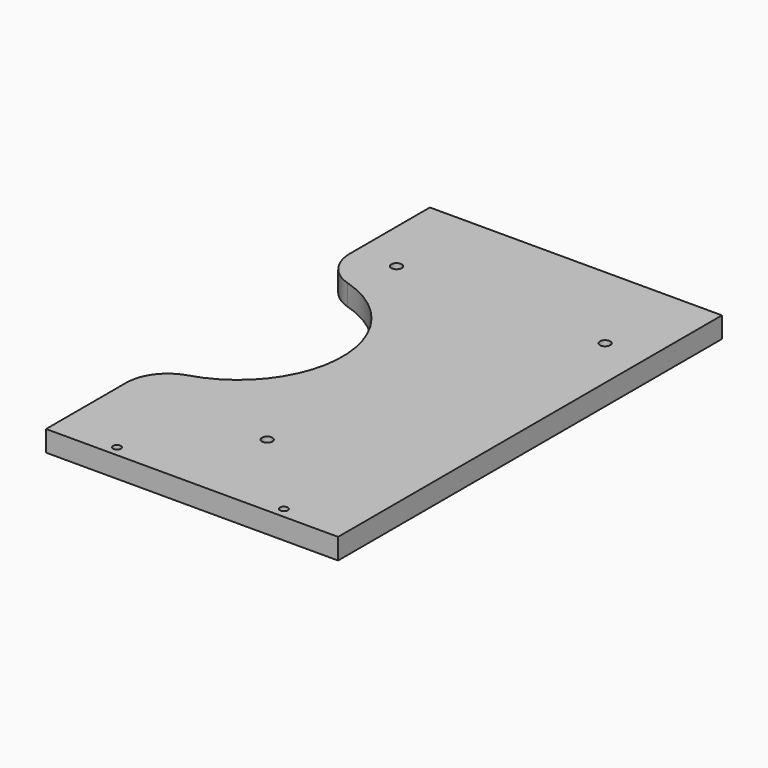
from build123d import *

# Parameters (mm, degrees)
F0_R     = 3.175
F1_DEPTH = 12.7
F2_R     = 25.4
F3_R     = 2.38125
F4_DEPTH = 12.701


with BuildPart() as f1:
    # F0 (on Top) → F1 (new body)
    with BuildSketch(Plane.XY):
        with BuildLine():
            Line((88.9, -146.05), (88.9, 146.05))
            Line((88.9, 146.05), (-88.9, 146.05))
            Line((-88.9, 146.05), (-88.9, 63.5))
            ThreePointArc((-88.9, 63.5), (-25.4, 0), (-88.9, -63.5))
            Line((-88.9, -63.5), (-88.9, -146.05))
            Line((-88.9, -146.05), (88.9, -146.05))
        make_face()
        with Locations((0, -88.9)):
            Circle(F0_R, mode=Mode.SUBTRACT)
        with Locations((-63.5, 88.9)):
            Circle(F0_R, mode=Mode.SUBTRACT)
        with Locations((63.5, 88.9)):
            Circle(F0_R, mode=Mode.SUBTRACT)
    extrude(amount=F1_DEPTH)

    # F2
    f2_edges = [f1.edges().sort_by_distance(p)[0] for p in [
        (-88.9, -63.5, 6.35),
        (-88.9, 63.5, 6.35),
    ]]
    fillet(f2_edges, radius=F2_R)

    # F3 (on face) → F4 (cut, through all)
    with BuildSketch(Plane.XY.offset(12.7)):
        with Locations((-50.8, -139.7)):
            Circle(F3_R)
        with Locations((50.8, -139.7)):
            Circle(F3_R)
    extrude(amount=-F4_DEPTH, mode=Mode.SUBTRACT)


solid = f1.part
